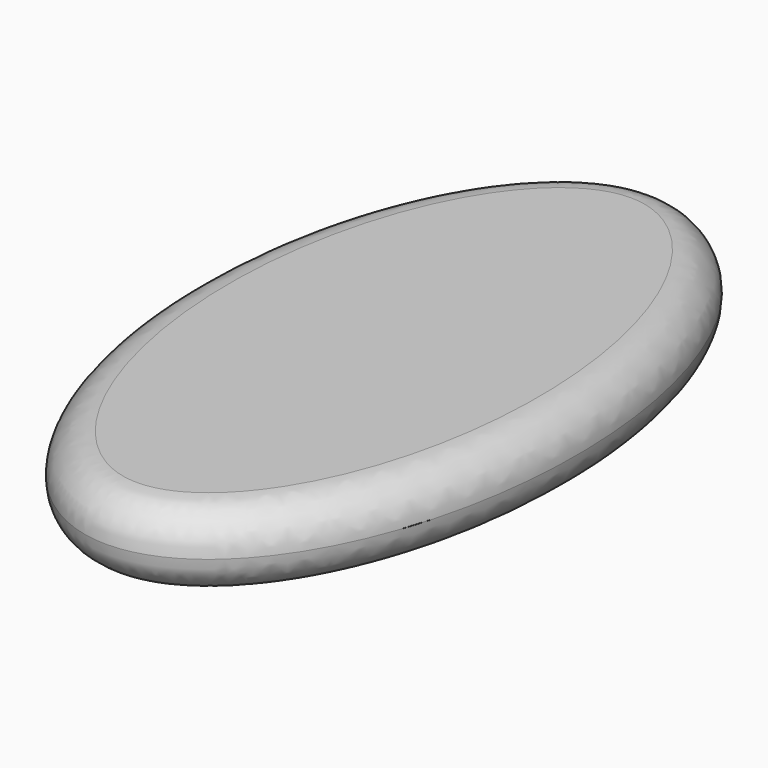
from build123d import *

# Parameters (mm, degrees)
F1_DEPTH = 50
F2_R     = 24.99999


# Not quite as in the source:
# - a fillet or chamfer is up to 0.001 mm smaller than in the source, because OpenCascade refuses the exact size


with BuildPart() as f1:
    # F0 (on Top) → F1 (new body)
    with BuildSketch(Plane.XY):
        with BuildLine():
            add(Edge.make_bspline(
                [(0, 225), (-216.5063509461, 225), (-108.2531754731, -112.5), (0, -450), (108.2531754731, -112.5), (216.5063509461, 225), (0, 225)],
                knots=[0, 0, 0, 2.0943951024, 2.0943951024, 4.1887902048, 4.1887902048, 6.2831853072, 6.2831853072, 6.2831853072], degree=2, weights=[1, 0.5, 1, 0.5, 1, 0.5, 1]))
        make_face()
    extrude(amount=F1_DEPTH)

    # F2 (radius 25 in the source; OpenCascade refuses exactly that, so slightly less here)
    f2_edges = [f1.edges().sort_by_distance(p)[0] for p in [
        (-7e-06, -225, 50),
        (-7e-06, -225, 0),
    ]]
    fillet(f2_edges, radius=F2_R)


solid = f1.part
